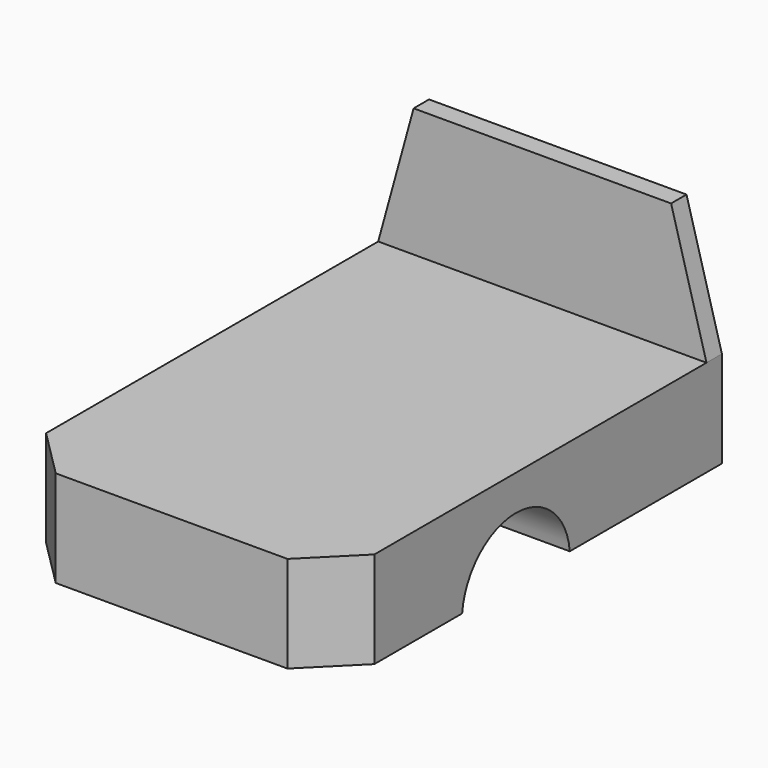
from build123d import *

# Parameters (mm, degrees)
F3_W          = 2590.8
F3_H          = 3810
F4_DEPTH      = 762
F5_R          = 533.4
F6_DEPTH      = 1295.401
F6_DEPTH_BACK = 1295.401
F8_DEPTH      = 762.001
F10_DEPTH     = 152.4


with BuildPart() as f4:
    # F3 (on Top) → F4 (new body)
    with BuildSketch(Plane.XY):
        with Locations((0, -1905)):
            Rectangle(F3_W, F3_H)
    extrude(amount=-F4_DEPTH)

    # F5 (on Right) → F6 (cut, two sides)
    with BuildSketch(Plane.YZ) as f6_sk:
        with Locations((-2032, -812.8)):
            Circle(F5_R)
    extrude(amount=-F6_DEPTH, mode=Mode.SUBTRACT)
    extrude(f6_sk.sketch, amount=F6_DEPTH_BACK, mode=Mode.SUBTRACT)

    # F7 (on Top) → F8 (cut, through all)
    with BuildSketch(Plane.XY):
        Polygon((1295.4, -3810), (1295.4, -3429), (914.4, -3810), align=None)
        Polygon((-1295.4, -3810), (-914.4, -3810), (-1295.4, -3429), align=None)
    extrude(amount=-F8_DEPTH, mode=Mode.SUBTRACT)

    # F9 (on Front) → F10 (join)
    with BuildSketch(Plane.XZ):
        Polygon((-1016, 1016), (-1295.4, 0), (1295.4, 0), (1016, 1016), align=None)
    extrude(amount=F10_DEPTH)


solid = f4.part
